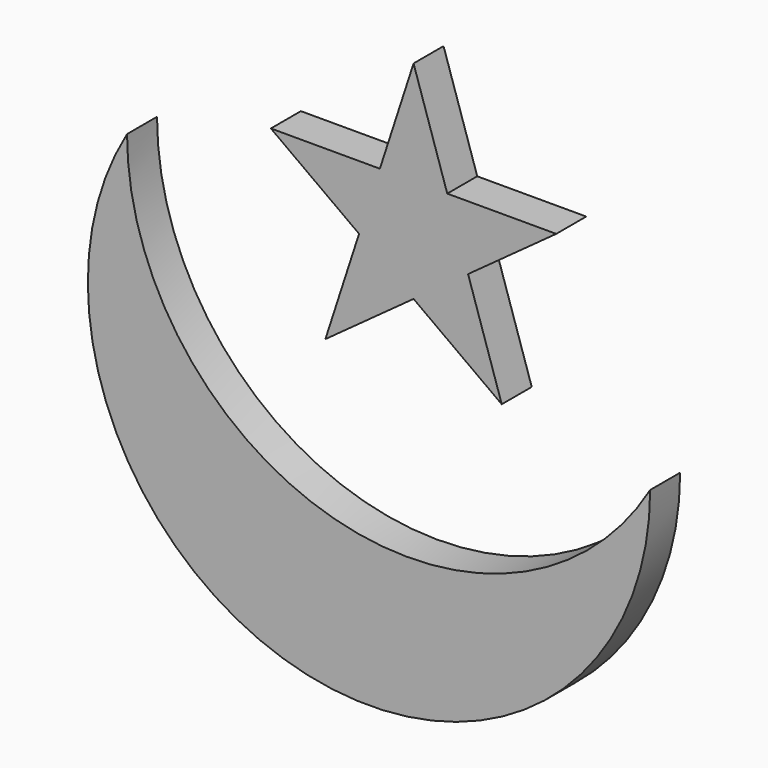
from build123d import *

# Parameters (mm, degrees)
F1_DEPTH = 2.54
F3_DEPTH = 2.54


with BuildPart() as f1:
    # F0 (on Front) → F1 (new body)
    with BuildSketch(Plane.XZ):
        with BuildLine():
            ThreePointArc((-16.3953601137, 9.7002405508), (-5.0284634748, -18.3743586305), (19.05, 0))
            ThreePointArc((19.05, 0), (-2.3738235885, -8.6741180797), (-16.3953601137, 9.7002405508))
        make_face()
    extrude(amount=F1_DEPTH)


with BuildPart() as f3:
    # F2 (on Front) → F3 (new body)
    with BuildSketch(Plane.XZ):
        Polygon((5.3014953599, 13.205398481), (3.0192455743, 20.2294410739), (0.7369957886, 13.205398481), align=None)
        Polygon((0.7369957886, 13.205398481), (-6.6485196593, 13.205398481), (-0.6735121497, 8.8643014201), align=None)
        Polygon((3.0192455743, 6.1813558881), (6.7120032982, 8.8643014201), (5.3014953599, 13.205398481), (0.7369957886, 13.205398481), (-0.6735121497, 8.8643014201), align=None)
        Polygon((6.7120032982, 8.8643014201), (12.6870108078, 13.205398481), (5.3014953599, 13.205398481), align=None)
        Polygon((3.0192455743, 6.1813558881), (8.9942530838, 1.8402588272), (6.7120032982, 8.8643014201), align=None)
        Polygon((-0.6735121497, 8.8643014201), (-2.9557619353, 1.8402588272), (3.0192455743, 6.1813558881), align=None)
    extrude(amount=F3_DEPTH)


solid = Compound([f1.part, f3.part])
